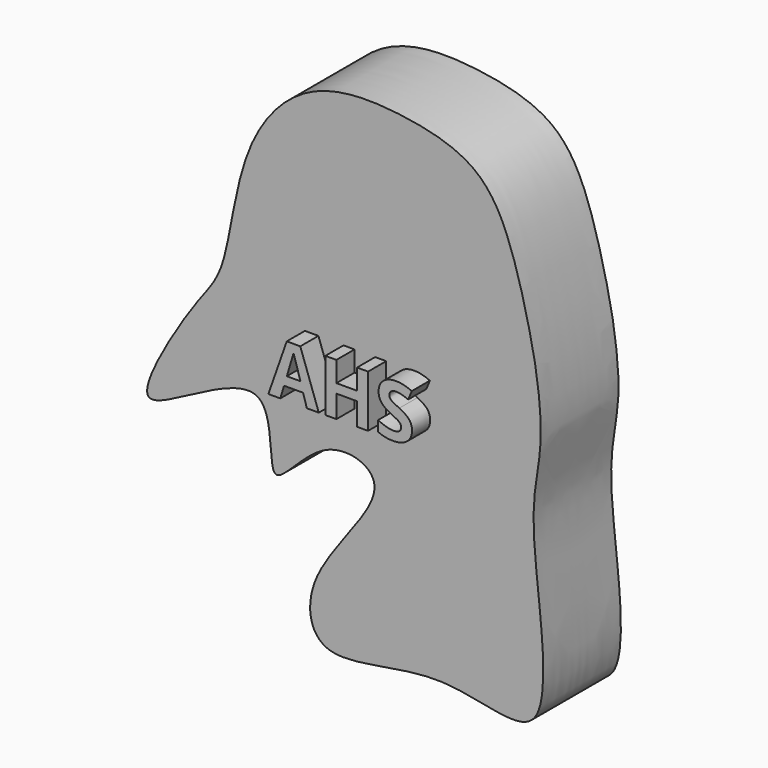
from build123d import *

# Parameters (mm, degrees)
F1_DEPTH     = 25.4
F2_TEXT_SIZE = 19.1213692435
F3_DEPTH     = 31.33283


# Not quite as in the source:
# - Text() gives the source's letters only with a copy of the font that has no kerning and outlines rounded to 1/6400 em; it was checked with that copy


with BuildPart() as f1:
    # F0 (on Front) → F1 (new body)
    with BuildSketch(Plane.XZ):
        with BuildLine():
            add(Edge.make_bspline(
                [(-64.2869178208, 37.2076611318), (-62.4361496686, 43.8616984619), (-60.3615602056, 66.0099679827), (-42.3584112508, 86.5144501599), (-17.2687522347, 85.8742634601), (2.3668547182, 80.7868009543), (10.8239385141, 66.2566566622), (15.6544460151, 46.7181562995), (17.4543222798, 38.1606202229), (19.7977635644, 19.7473015814), (13.8365807497, 3.2713693166), (25.8072959997, -53.8492198893), (-7.9179196613, -36.9352820971), (-40.5200906707, -50.4769156607), (-44.4931994061, -26.7273541181), (-15.9670612166, -1.2007062503), (-39.2047282352, 6.3675698747), (-54.5631197704, -18.5147345546), (-48.6327094528, 21.9871355325), (-96.1437679252, -15.6822900082), (-73.2225199932, 22.9160269622), (-67.982313347, 28.8031713378), (-65.3158410228, 33.5083898927), (-64.2869178208, 37.2076611318)],
                knots=[0, 0, 0, 0, 0.0560486891, 0.1092726092, 0.1607754132, 0.2070836249, 0.24957684, 0.2963638108, 0.3285716753, 0.3714200175, 0.419530475, 0.4894058672, 0.5414960445, 0.5997778721, 0.6412133647, 0.6997948541, 0.7382795094, 0.7812297853, 0.8249292681, 0.8823986711, 0.9346829805, 0.9688400751, 1, 1, 1, 1], degree=3))
        make_face()
    extrude(amount=F1_DEPTH)

    # F2 (on Front) → F3 (join)
    with BuildSketch(Plane.XZ):
        with Locations((-47.9479015339, 13.499982655)):
            Text('AHS', F2_TEXT_SIZE, font='Open Sans', font_style=FontStyle.BOLD, text_align=(TextAlign.LEFT, TextAlign.BOTTOM))
    extrude(amount=F3_DEPTH)


solid = f1.part
